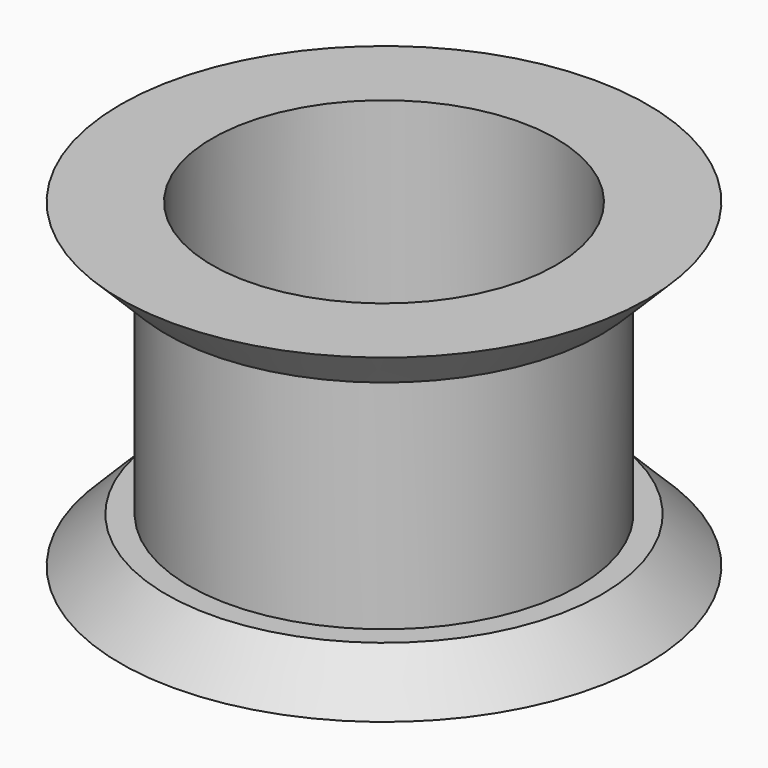
from build123d import *

# Parameters (mm, degrees)
F0_R     = 8.5
F1_DEPTH = 14
F2_R     = 11.5
F2_R_2   = 8.5
F4_DEPTH = 2
F5_SIZE  = 1.99999
F3_R     = 11.5
F3_R_2   = 8.5
F6_DEPTH = 2
F7_SIZE  = 1.99999
F8_R     = 7.5
F9_DEPTH = 14.001


# Not quite as in the source:
# - a fillet or chamfer is up to 0.001 mm smaller than in the source, because OpenCascade refuses the exact size


with BuildPart() as f1:
    # F0 (on Top) → F1 (new body)
    with BuildSketch(Plane.XY):
        Circle(F0_R)
    extrude(amount=F1_DEPTH)

    # F2 (on face) → F4 (join)
    with BuildSketch(Plane.XY.offset(14)):
        Circle(F2_R)
        Circle(F2_R_2, mode=Mode.SUBTRACT)
    extrude(amount=-F4_DEPTH)

    # F5 (size 2 in the source; OpenCascade refuses exactly that, so slightly less here)
    f5_edges = [f1.edges().sort_by_distance(p)[0] for p in [
        (-11.5, 0, 12),
    ]]
    chamfer(f5_edges, length=F5_SIZE)

    # F3 (on face) → F6 (join)
    with BuildSketch(Plane(origin=(0, 0, 0), x_dir=(1, 0, 0), z_dir=(0, 0, -1))):
        Circle(F3_R)
        Circle(F3_R_2, mode=Mode.SUBTRACT)
    extrude(amount=-F6_DEPTH)

    # F7 (size 2 in the source; OpenCascade refuses exactly that, so slightly less here)
    f7_edges = [f1.edges().sort_by_distance(p)[0] for p in [
        (-11.5, 0, 2),
    ]]
    chamfer(f7_edges, length=F7_SIZE)

    # F8 (on face) → F9 (cut, through all)
    with BuildSketch(Plane.XY.offset(14)):
        Circle(F8_R)
    extrude(amount=-F9_DEPTH, mode=Mode.SUBTRACT)


solid = f1.part
